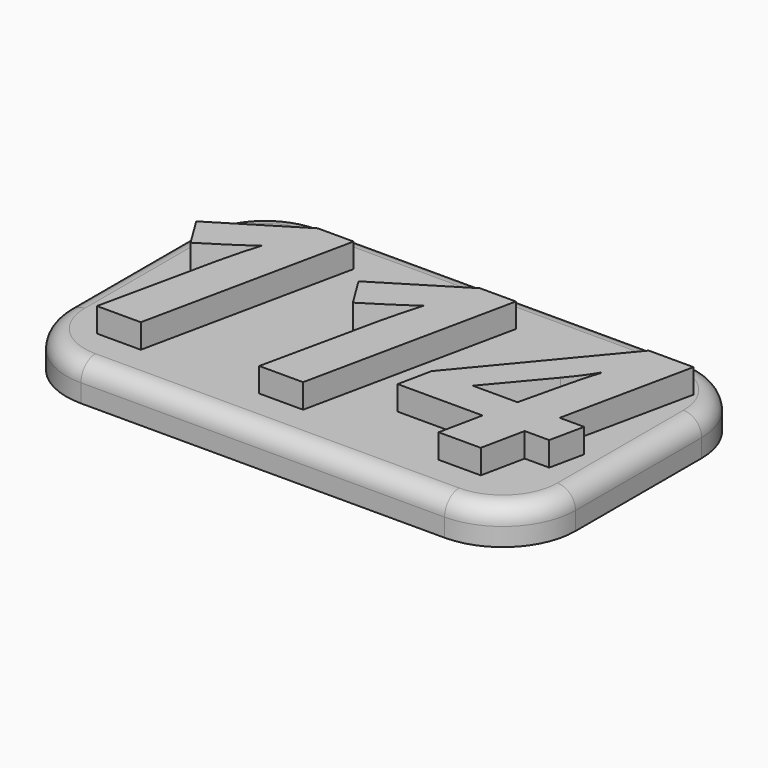
from build123d import *

# Parameters (mm, degrees)
F0_W         = 42
F0_H         = 25
F1_DEPTH     = 3
F2_R         = 6
F3_R         = 1.5
F4_TEXT_SIZE = 24.3055555556
F5_DEPTH     = 2


# Not quite as in the source:
# - Text() gives the source's letters only with a copy of the font that has no kerning and outlines rounded to 1/6400 em; it was checked with that copy


with BuildPart() as f1:
    # F0 (on Top) → F1 (new body)
    with BuildSketch(Plane.XY):
        Rectangle(F0_W, F0_H)
    extrude(amount=F1_DEPTH)

    # F2
    f2_edges = [f1.edges().sort_by_distance(p)[0] for p in [
        (-21, -12.5, 1.5),
        (21, -12.5, 1.5),
        (-21, 12.5, 1.5),
        (21, 12.5, 1.5),
    ]]
    fillet(f2_edges, radius=F2_R)

    # F3
    f3_edges = [f1.edges().sort_by_distance(p)[0] for p in [
        (0, -12.5, 3),
    ]]
    fillet(f3_edges, radius=F3_R)

    # F4 (on face) → F5 (join)
    with BuildSketch(Plane.XY.offset(3)):
        with Locations((-21.2261827257, -8.75)):
            Text('114', F4_TEXT_SIZE, font='Open Sans', font_style=FontStyle.BOLDITALIC, text_align=(TextAlign.LEFT, TextAlign.BOTTOM))
    extrude(amount=F5_DEPTH)


solid = f1.part
